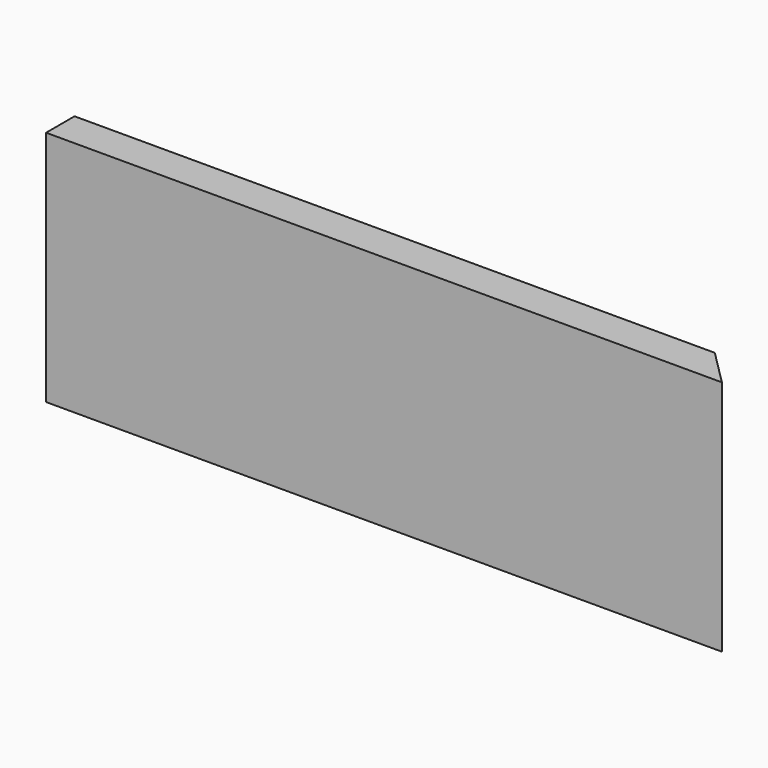
from build123d import *

# Parameters (mm, degrees)
F0_W     = 361.95
F0_H     = 127
F1_DEPTH = 19.05
F2_SIZE2 = 19.04999
F2_SIZE  = 19.04999


# Not quite as in the source:
# - a fillet or chamfer is up to 0.001 mm smaller than in the source, because OpenCascade refuses the exact size


with BuildPart() as f1:
    # F0 (on Front) → F1 (new body)
    with BuildSketch(Plane.XZ):
        with Locations((29.6110501051, 33.5559173692)):
            Rectangle(F0_W, F0_H)
    extrude(amount=F1_DEPTH)

    # F2 (size 19.05 and 19.05 in the source; OpenCascade refuses exactly that, so slightly less here)
    f2_edges = [f1.edges().sort_by_distance(p)[0] for p in [
        (210.58605, 0, 33.555917),
    ]]
    chamfer(f2_edges, length=F2_SIZE, length2=F2_SIZE2)


solid = f1.part
